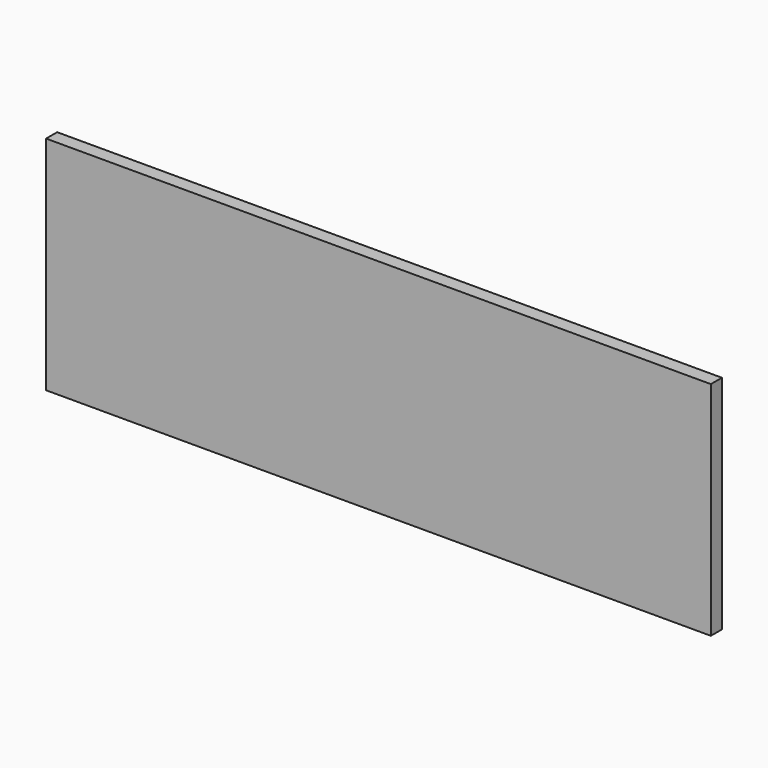
from build123d import *

# Parameters (mm, degrees)
F0_W     = 304.8
F0_H     = 101.6
F1_DEPTH = 6.35


# Not quite as in the source:
# - a length typed as a fraction of an inch, garbled in the dataset ("3 / 203.2 mm" for 3/8 in), is restored


with BuildPart() as f1:
    # F0 (on Front) → F1 (new body)
    with BuildSketch(Plane.XZ):
        Rectangle(F0_W, F0_H)
    extrude(amount=F1_DEPTH)


solid = f1.part
